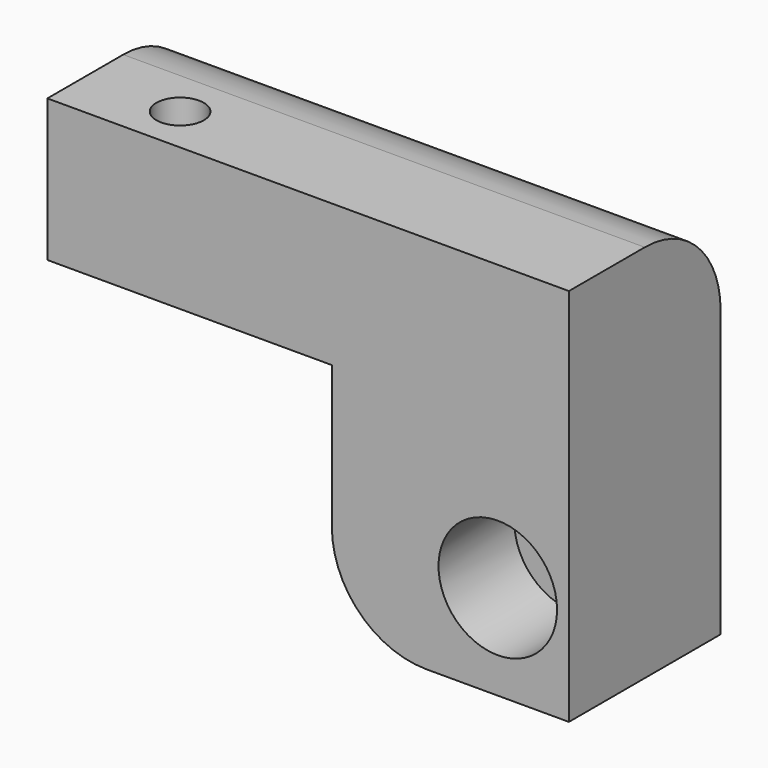
from build123d import *

# Parameters (mm, degrees)
F0_R           = 15.875
F0_W           = 76.2
F0_H           = 69.85
F1_DEPTH       = 50.8
F2_R           = 25.4
F3_R           = 25.4
F5_SIZE2       = 31.743353
F5_SIZE        = 50.79999
F7_D           = 12.7
F8_D           = 19.05
F8_CBORE_D     = 31.75
F8_CBORE_DEPTH = 25.4


# Not quite as in the source:
# - a fillet or chamfer is up to 0.001 mm smaller than in the source, because OpenCascade refuses the exact size


with BuildPart() as f1:
    # F0 (on Front) → F1 (new body)
    with BuildSketch(Plane.XZ):
        Polygon((65.6778021347, 50.8), (2.1778021347, 50.8), (2.1778021347, -19.05), (2.1778021347, -50.8), (65.6778021347, -50.8), align=None)
        with Locations((46.6278021347, -25.4)):
            Circle(F0_R, mode=Mode.SUBTRACT)
        with Locations((46.6278021347, -25.4)):
            Circle(F0_R)
        with Locations((-35.9221978653, 15.875)):
            Rectangle(F0_W, F0_H)
    extrude(amount=F1_DEPTH)

    # F2
    f2_edges = [f1.edges().sort_by_distance(p)[0] for p in [
        (2.177802, -25.4, -50.8),
    ]]
    fillet(f2_edges, radius=F2_R)

    # F3
    f3_edges = [f1.edges().sort_by_distance(p)[0] for p in [
        (-4.172198, 0, 50.8),
    ]]
    fillet(f3_edges, radius=F3_R)

    # F5 (size 50.8 and 31.743363077 in the source; OpenCascade refuses exactly that, so slightly less here)
    f5_edges = [f1.edges().sort_by_distance(p)[0] for p in [
        (-35.922198, -50.8, -19.05),
    ]]
    f5_side = f1.faces().sort_by_distance((-35.922198, -25.4, -19.05))[0]
    chamfer(f5_edges, length=F5_SIZE, length2=F5_SIZE2, reference=f5_side)

    # F7 (through all)
    with Locations(Plane.XY.offset(50.8)):
        with Locations((-48.6221978653, -38.1)):
            Hole(F7_D / 2)

    # F8 (through all)
    with Locations(Plane.XZ.offset(50.8)):
        with Locations((46.6278021347, -25.4)):
            CounterBoreHole(F8_D / 2, F8_CBORE_D / 2, F8_CBORE_DEPTH)


solid = f1.part
